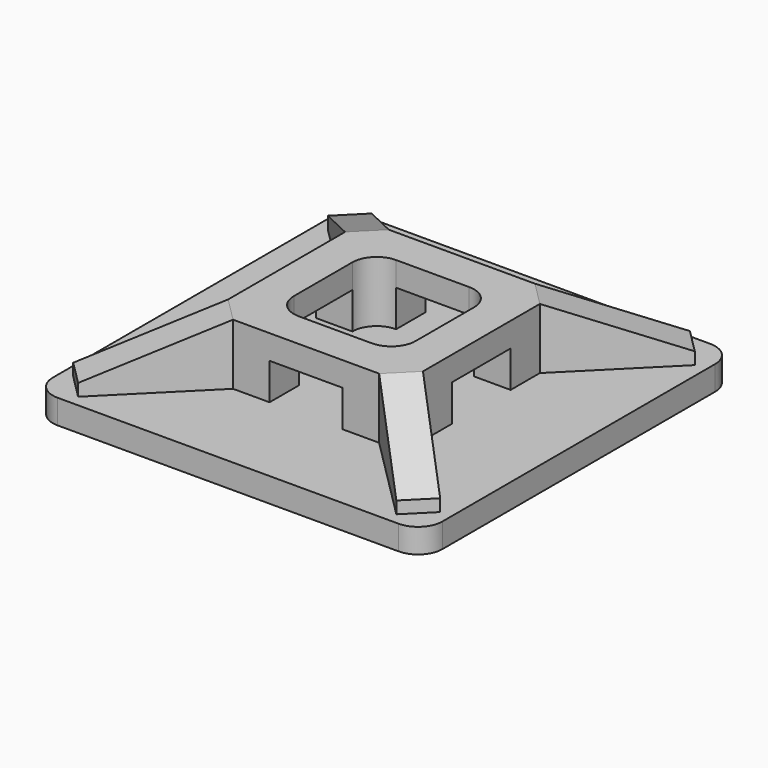
from build123d import *

# Parameters (mm, degrees)
F0_W           = 16
F0_H           = 16
F1_DEPTH       = 1
F2_W           = 8
F2_H           = 8
F2_W_2         = 5
F2_H_2         = 5
F3_DEPTH       = 2.5
F4_SIZE        = 1
F5_DEPTH       = 5
F6_DEPTH       = 5
F7_DEPTH       = 5
F8_DEPTH       = 5
F9_SIZE2       = 2
F9_SIZE        = 5
F10_W          = 3
F10_H          = 1.5
F11_DEPTH      = 8.001
F11_DEPTH_BACK = 8.001
F12_W          = 3
F12_H          = 1.5
F13_DEPTH      = 8.001
F13_DEPTH_BACK = 8.001
F14_R          = 1


with BuildPart() as f1:
    # F0 (on Top) → F1 (new body)
    with BuildSketch(Plane.XY):
        Rectangle(F0_W, F0_H)
    extrude(amount=F1_DEPTH)

    # F2 (on face) → F3 (join)
    with BuildSketch(Plane.XY.offset(1)):
        Rectangle(F2_W, F2_H)
        Rectangle(F2_W_2, F2_H_2, mode=Mode.SUBTRACT)
    extrude(amount=F3_DEPTH)

    # F4
    f4_edges = [f1.edges().sort_by_distance(p)[0] for p in [
        (4, 4, 2.25),
        (-4, 4, 2.25),
        (-4, -4, 2.25),
        (4, -4, 2.25),
    ]]
    chamfer(f4_edges, length=F4_SIZE)

    # F5 (add): a face of the model
    f5_faces = [f1.faces().sort_by_distance(p)[0] for p in [
        (-3.5, -3.5, 2.25),
    ]]
    extrude(f5_faces, amount=F5_DEPTH)

    # F6 (add): a face of the model
    f6_faces = [f1.faces().sort_by_distance(p)[0] for p in [
        (3.5, -3.5, 2.25),
    ]]
    extrude(f6_faces, amount=F6_DEPTH)

    # F7 (add): a face of the model
    f7_faces = [f1.faces().sort_by_distance(p)[0] for p in [
        (-3.5, 3.5, 2.25),
    ]]
    extrude(f7_faces, amount=F7_DEPTH)

    # F8 (add): a face of the model
    f8_faces = [f1.faces().sort_by_distance(p)[0] for p in [
        (3.5, 3.5, 2.25),
    ]]
    extrude(f8_faces, amount=F8_DEPTH)

    # F9
    f9_edges = [f1.edges().sort_by_distance(p)[0] for p in [
        (-7.035534, 7.035534, 3.5),
        (-7.035534, -7.035534, 3.5),
        (7.035534, -7.035534, 3.5),
        (7.035534, 7.035534, 3.5),
    ]]
    f9_side = f1.faces().sort_by_distance((0, 3.786863, 3.5))[0]
    chamfer(f9_edges, length=F9_SIZE, length2=F9_SIZE2, reference=f9_side)

    # F10 (on Front) → F11 (cut, two sides)
    with BuildSketch(Plane.XZ) as f11_sk:
        with Locations((0, 1.75)):
            Rectangle(F10_W, F10_H)
    extrude(amount=-F11_DEPTH, mode=Mode.SUBTRACT)
    extrude(f11_sk.sketch, amount=F11_DEPTH_BACK, mode=Mode.SUBTRACT)

    # F12 (on Right) → F13 (cut, two sides)
    with BuildSketch(Plane.YZ) as f13_sk:
        with Locations((0, 1.75)):
            Rectangle(F12_W, F12_H)
    extrude(amount=-F13_DEPTH, mode=Mode.SUBTRACT)
    extrude(f13_sk.sketch, amount=F13_DEPTH_BACK, mode=Mode.SUBTRACT)

    # F14
    f14_edges = [f1.edges().sort_by_distance(p)[0] for p in [
        (-2.5, 2.5, 2.25),
        (-2.5, -2.5, 2.25),
        (2.5, 2.5, 2.25),
        (2.5, -2.5, 2.25),
        (8, -8, 0.5),
        (8, 8, 0.5),
        (-8, -8, 0.5),
        (-8, 8, 0.5),
    ]]
    fillet(f14_edges, radius=F14_R)


solid = f1.part
